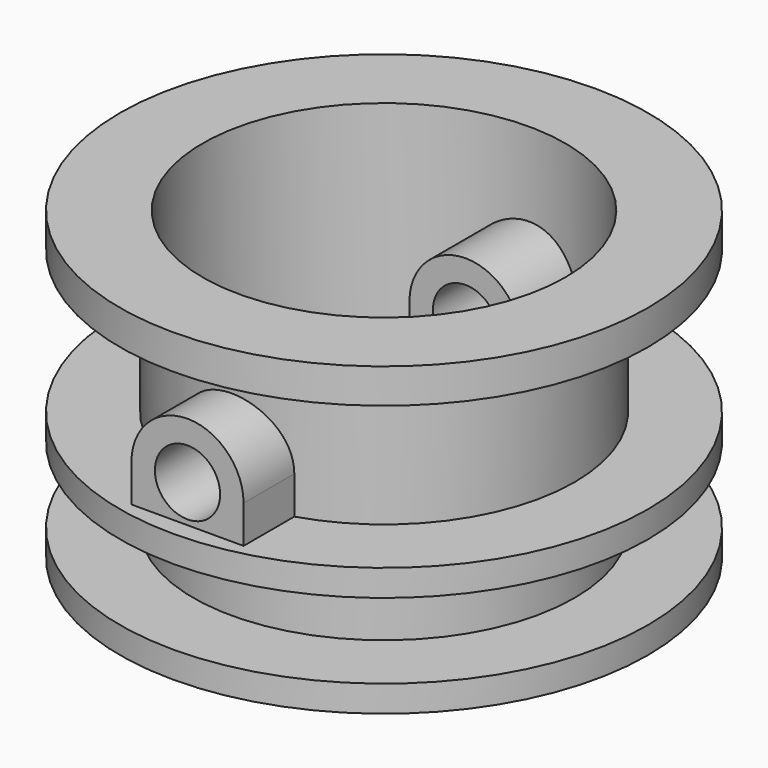
from build123d import *

# Parameters (mm, degrees)
F2_R      = 8.9
F3_DEPTH  = 1.3
F4_R      = 8.9
F5_DEPTH  = 12.8
F7_START  = 5
F7_DEPTH  = 7.05
F9_START  = 5
F8_W      = 5.5
F8_H      = 1.3
F8_H_2    = 3.7
F9_DEPTH  = 3.5
F10_R     = 1.6
F11_DEPTH = 7.05
F12_W     = 3.1
F12_H     = 2.8
F13_DEPTH = 3.5


# Not quite as in the source:
# - a feature of the source that left no trace in its solid (it failed there, or was rolled back) is left out
# - a pattern or mirror of a feature is missing from the dataset's text; its kind, count and spacing are read off the source's solid


with BuildPart() as f1:
    # F0 (on Front) → F1 (revolve)
    with BuildSketch(Plane.XZ):
        Polygon((-12.95, 0), (0, 0), (0, 15), (-12.95, 15), (-12.95, 13.3), (-9.35, 13.3), (-9.35, 6.3), (-12.95, 6.3), (-12.95, 5), (-9.35, 5), (-9.35, 1.3), (-12.95, 1.3), align=None)
    revolve(axis=Axis((0, 0, 7.5), (0, 0, -1)))

    # F2 (on face) → F3 (cut)
    with BuildSketch(Plane(origin=(0, 0, 0), x_dir=(1, 0, 0), z_dir=(0, 0, -1))):
        Circle(F2_R)
    extrude(amount=-F3_DEPTH, mode=Mode.SUBTRACT)

    # F4 (on face) → F5 (cut)
    with BuildSketch(Plane.XY.offset(15)):
        Circle(F4_R)
    extrude(amount=-F5_DEPTH, mode=Mode.SUBTRACT)

    # F6 (on Front) → F7 (join)
    with BuildSketch(Plane.XZ.offset(F7_START)):
        with BuildLine():
            Line((2.75, 6.3), (2.75, 8.15))
            ThreePointArc((2.75, 8.15), (0, 10.9), (-2.75, 8.15))
            Line((-2.75, 8.15), (-2.75, 6.3))
            Line((-2.75, 6.3), (2.75, 6.3))
        make_face()
    f7 = extrude(amount=F7_DEPTH)

    # F7_copies: F7 across plane
    add(f7.mirror(Plane.ZX))

    # F8 (on Front) → F9 (join)
    with BuildSketch(Plane.XZ.offset(F9_START)):
        with BuildLine():
            ThreePointArc((2.75, 8.15), (0, 10.9), (-2.75, 8.15))
            Line((-2.75, 8.15), (-2.75, 6.3))
            Line((-2.75, 6.3), (2.75, 6.3))
            Line((2.75, 6.3), (2.75, 8.15))
        make_face()
        with Locations((0, 5.65)):
            Rectangle(F8_W, F8_H)
        with Locations((0, 3.15)):
            Rectangle(F8_W, F8_H_2)
    f9 = extrude(amount=F9_DEPTH)

    # F9_copies: F9 across plane
    add(f9.mirror(Plane.ZX))

    # F10 (on face) → F11 (cut, through all)
    with BuildSketch(Plane.XZ.offset(12.05)):
        with Locations((0, 8.15)):
            Circle(F10_R)
    f11 = extrude(amount=-F11_DEPTH, mode=Mode.SUBTRACT)

    # F11_copies: F11 across plane
    add(f11.mirror(Plane.ZX), mode=Mode.SUBTRACT)

    # F12 (on face) → F13 (cut)
    with BuildSketch(Plane(origin=(0, 0, 1.3), x_dir=(1, 0, 0), z_dir=(0, 0, -1))):
        with Locations((0, 7.3639888179)):
            Rectangle(F12_W, F12_H)
    f13 = extrude(amount=-F13_DEPTH, mode=Mode.SUBTRACT)

    # F13_copies: F13 across plane
    add(f13.mirror(Plane.ZX), mode=Mode.SUBTRACT)


solid = f1.part
